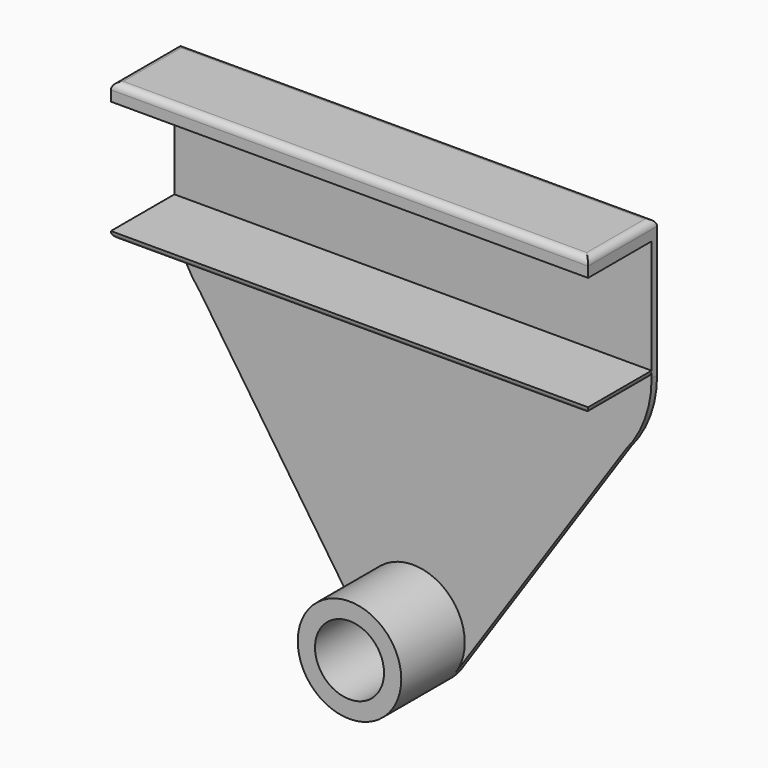
from build123d import *

# Parameters (mm, degrees)
F0_W     = 138.2855419193
F0_H     = 33
F0_R     = 10
F0_H_2   = 5
F0_H_3   = 2
F1_DEPTH = 2
F2_DEPTH = 25
F3_R     = 1.99999


# Not quite as in the source:
# - a fillet or chamfer is up to 0.001 mm smaller than in the source, because OpenCascade refuses the exact size


with BuildPart() as f1:
    # F0 (on Front) → F1 (new body)
    with BuildSketch(Plane.XZ):
        with BuildLine():
            ThreePointArc((61.670333147, -40.4906272888), (67.2163679442, -30.9053098713), (69.1427709597, -20))
            Line((69.1427709597, -20), (-69.1427709597, -20))
            ThreePointArc((-69.1427709597, -20), (-67.2163679442, -30.9053098713), (-61.670333147, -40.4906272888))
            Line((-61.670333147, -40.4906272888), (-12.4304277098, -113.3955027814))
            ThreePointArc((-12.4304277098, -113.3955027814), (-4.3899649403, -90.6567713599), (15, -105))
            ThreePointArc((15, -105), (14.3432286401, -109.3899649403), (12.4304277098, -113.3955027814))
            Line((12.4304277098, -113.3955027814), (61.670333147, -40.4906272888))
        make_face()
        with Locations((0, -1.5)):
            Rectangle(F0_W, F0_H)
        with BuildLine():
            ThreePointArc((-12.4304277098, -113.3955027814), (0, -120), (12.4304277098, -113.3955027814))
            ThreePointArc((12.4304277098, -113.3955027814), (14.3432286401, -109.3899649403), (15, -105))
            ThreePointArc((15, -105), (-4.3899649403, -90.6567713599), (-12.4304277098, -113.3955027814))
        make_face()
        with Locations((0, -105)):
            Circle(F0_R, mode=Mode.SUBTRACT)
        with Locations((0, 17.5)):
            Rectangle(F0_W, F0_H_2)
        with Locations((0, -105)):
            Circle(F0_R)
        with Locations((0, -19)):
            Rectangle(F0_W, F0_H_3)
    extrude(amount=F1_DEPTH)

    # F0 (on Front) → F2 (join)
    with BuildSketch(Plane.XZ):
        with Locations((0, 17.5)):
            Rectangle(F0_W, F0_H_2)
        with Locations((0, -19)):
            Rectangle(F0_W, F0_H_3)
        with BuildLine():
            ThreePointArc((-12.4304277098, -113.3955027814), (0, -120), (12.4304277098, -113.3955027814))
            ThreePointArc((12.4304277098, -113.3955027814), (14.3432286401, -109.3899649403), (15, -105))
            ThreePointArc((15, -105), (-4.3899649403, -90.6567713599), (-12.4304277098, -113.3955027814))
        make_face()
        with Locations((0, -105)):
            Circle(F0_R, mode=Mode.SUBTRACT)
    extrude(amount=F2_DEPTH)

    # F3 (radius 2 in the source; OpenCascade refuses exactly that, so slightly less here)
    f3_edges = [f1.edges().sort_by_distance(p)[0] for p in [
        (69.142771, -12.5, 20),
        (0, -25, 20),
        (-69.142771, -12.5, 20),
        (0, 0, 20),
        (0, -25, -20),
        (69.142771, -13.5, -20),
        (-69.142771, -13.5, -20),
    ]]
    fillet(f3_edges, radius=F3_R)


solid = f1.part
